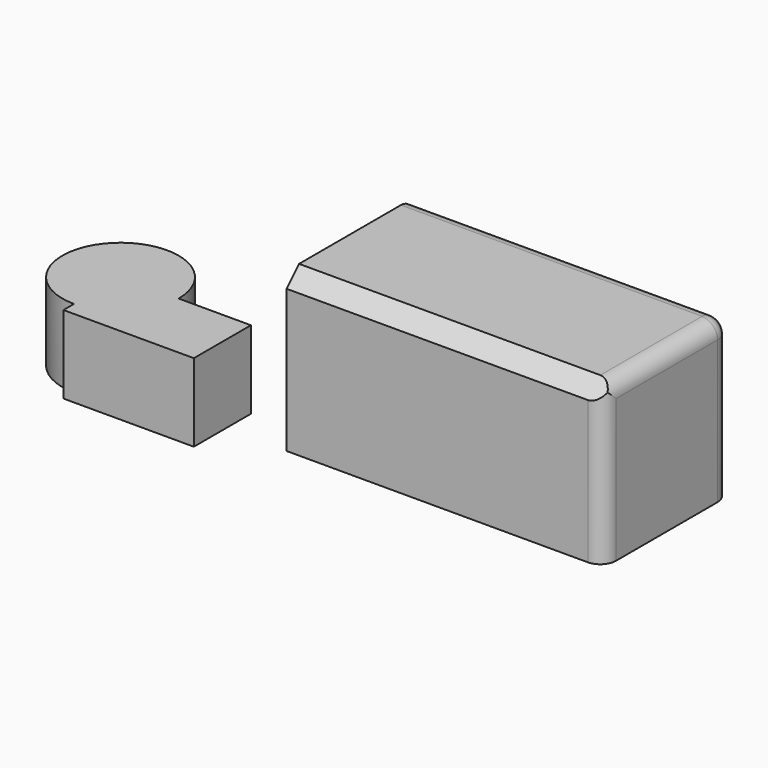
from build123d import *

# Parameters (mm, degrees)
F0_W     = 101.6
F0_H     = 50.8
F1_DEPTH = 50.8
F2_R     = 5.08
F4_DEPTH = 25
F5_SIZE  = 5
F6_R     = 5
F7_R     = 4.99999


# Not quite as in the source:
# - a fillet or chamfer is up to 0.001 mm smaller than in the source, because OpenCascade refuses the exact size


with BuildPart() as f1:
    # F0 (on Top) → F1 (new body)
    with BuildSketch(Plane.XY):
        with Locations((50.8, -25.4)):
            Rectangle(F0_W, F0_H)
    extrude(amount=F1_DEPTH)

    # F2
    f2_edges = [f1.edges().sort_by_distance(p)[0] for p in [
        (101.6, 0, 25.4),
    ]]
    fillet(f2_edges, radius=F2_R)

    # F5
    f5_edges = [f1.edges().sort_by_distance(p)[0] for p in [
        (50.8, -50.8, 50.8),
    ]]
    chamfer(f5_edges, length=F5_SIZE)

    # F6
    f6_edges = [f1.edges().sort_by_distance(p)[0] for p in [
        (48.26, 0, 50.8),
    ]]
    fillet(f6_edges, radius=F6_R)

    # F7 (radius 5 in the source; OpenCascade refuses exactly that, so slightly less here)
    f7_edges = [f1.edges().sort_by_distance(p)[0] for p in [
        (101.6, -50.8, 22.9),
    ]]
    fillet(f7_edges, radius=F7_R)


with BuildPart() as f4:
    # F3 (on Top) → F4 (new body)
    with BuildSketch(Plane.XY):
        with BuildLine():
            Line((-61.385255307, -59.2657432558), (-61.385255307, -40.6210906804))
            Line((-61.385255307, -40.6210906804), (-42.7406027316, -40.6210906804))
            ThreePointArc((-42.7406027316, -40.6210906804), (-74.5690155759, -27.4373304114), (-61.385255307, -59.2657432558))
        make_face()
        with BuildLine():
            Line((-42.7406027316, -40.6210906804), (-61.385255307, -40.6210906804))
            Line((-61.385255307, -40.6210906804), (-61.385255307, -59.2657432558))
            ThreePointArc((-61.385255307, -59.2657432558), (-48.201495038, -53.8048509493), (-42.7406027316, -40.6210906804))
        make_face()
        with BuildLine():
            Line((-19.57654953, -40.6210906804), (-42.7406027316, -40.6210906804))
            ThreePointArc((-42.7406027316, -40.6210906804), (-48.201495038, -53.8048509493), (-61.385255307, -59.2657432558))
            Line((-61.385255307, -59.2657432558), (-61.385255307, -63.4969770908))
            Line((-61.385255307, -63.4969770908), (-19.57654953, -63.4969770908))
            Line((-19.57654953, -63.4969770908), (-19.57654953, -40.6210906804))
        make_face()
    extrude(amount=F4_DEPTH)


solid = Compound([f1.part, f4.part])
